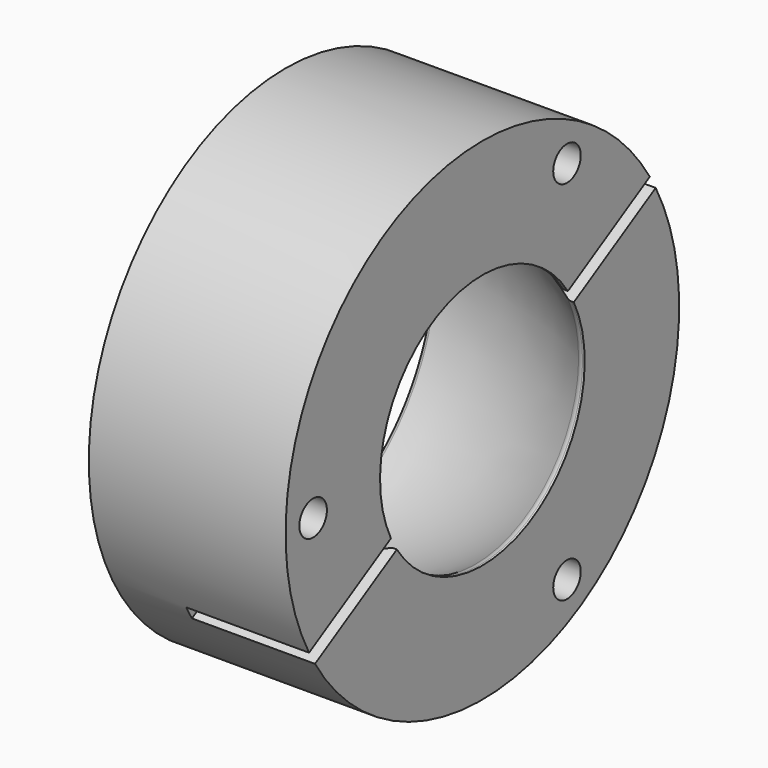
from build123d import *

# Parameters (mm, degrees)
F3_R            = 1
F4_R            = 3.5
F5_DEPTH        = 40.001
F5_COPIES_COUNT = 3
F7_DEPTH        = 25


# Not quite as in the source:
# - a fillet or chamfer that OpenCascade refuses, or shapes differently, is made with other operations: its cross-section is extruded or revolved along the edge and cut away or added
# - a pattern or mirror of a feature is missing from the dataset's text; its kind, count and spacing are read off the source's solid


with BuildPart() as f1:
    # F0 (on Front) → F1 (revolve)
    with BuildSketch(Plane.XZ):
        with BuildLine():
            Line((40, 50), (0, 50))
            Line((0, 50), (0, 37))
            ThreePointArc((0, 37), (20.2607995894, 34.1973803623), (39, 26))
            Line((39, 26), (40, 26))
            Line((40, 26), (40, 50))
        make_face()
    revolve(axis=Axis((-20.2939212322, 0, 0), (-1, 0, 0)))

    # F2: fillet of radius 2 on 1 edges, made by hand

    # F2_s1 → F2_t2 (revolve, cut)
    with BuildSketch(Plane.XZ):
        with BuildLine():
            ThreePointArc((39.5600808897, 26), (39.0242917631, 26.0731035285), (38.5276707123, 26.2870699881))
            ThreePointArc((38.5276707123, 26.2870699881), (38.7641010964, 26.1439722286), (39, 26))
            Line((39, 26), (39.5600808897, 26))
        make_face()
    revolve(axis=Axis((39, 0, 0), (-1, 0, 0)), mode=Mode.SUBTRACT)

    # F3
    f3_edges = [f1.edges().sort_by_distance(p)[0] for p in [
        (0, 0, -37),
    ]]
    fillet(f3_edges, radius=F3_R)

    # F4 (on face) → F5 (cut, through all)
    with BuildSketch(Plane(origin=(0, 0, 0), x_dir=(0, -1, 0), z_dir=(-1, 0, 0))):
        with Locations((43, 0)):
            Circle(F4_R)
    f5 = extrude(amount=-F5_DEPTH, mode=Mode.SUBTRACT)

    # F5_copies: F5 ×3 about axis
    f5_copies_axis = Axis((0, 0, 0), (1, 0, 0))
    for i in range(1, F5_COPIES_COUNT):
        add(f5.rotate(f5_copies_axis, i * 360 / F5_COPIES_COUNT), mode=Mode.SUBTRACT)

    # F6 (on face) → F7 (cut)
    with BuildSketch(Plane.YZ.offset(40)):
        with BuildLine():
            ThreePointArc((44.0317802314, 23.6897093619), (43.3012701892, 25), (42.5317802314, 26.2877855733))
            Line((42.5317802314, 26.2877855733), (21.7291570127, 14.2773854581))
            ThreePointArc((21.7291570127, 14.2773854581), (22.5166604984, 13), (23.2291570127, 11.6793092467))
            Line((23.2291570127, 11.6793092467), (44.0317802314, 23.6897093619))
        make_face()
        with BuildLine():
            Line((-23.2291570127, -11.6793092467), (-44.0317802314, -23.6897093619))
            ThreePointArc((-44.0317802314, -23.6897093619), (-43.3012701892, -25), (-42.5317802314, -26.2877855733))
            Line((-42.5317802314, -26.2877855733), (-21.7291570127, -14.2773854581))
            ThreePointArc((-21.7291570127, -14.2773854581), (-22.5166604984, -13), (-23.2291570127, -11.6793092467))
        make_face()
    extrude(amount=-F7_DEPTH, mode=Mode.SUBTRACT)


solid = f1.part
